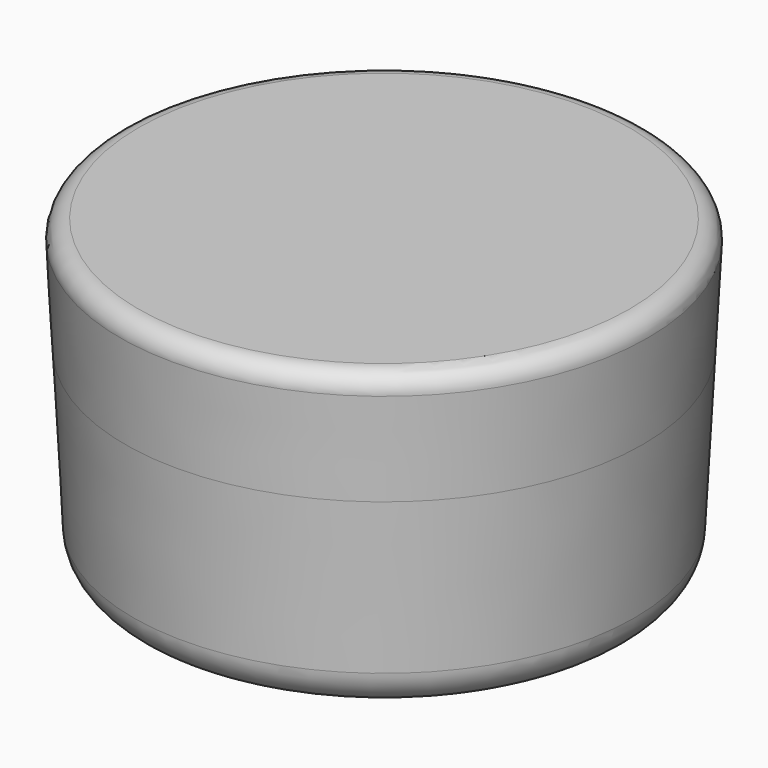
from build123d import *

# Parameters (mm, degrees)
F0_R     = 32.5
F1_DEPTH = 25
F1_TAPER = -3
F2_R     = 33.8101944821
F3_DEPTH = 15
F3_TAPER = -3
F4_R     = 2.4
F5_R     = 5


with BuildPart() as f1:
    # F0 (on Top) → F1 (new body)
    with BuildSketch(Plane.XY):
        Circle(F0_R)
    extrude(amount=F1_DEPTH, taper=F1_TAPER)

    # F5
    f5_edges = [f1.edges().sort_by_distance(p)[0] for p in [
        (-32.5, 0, 0),
    ]]
    fillet(f5_edges, radius=F5_R)


with BuildPart() as f3:
    # F2 (on face) → F3 (new body)
    with BuildSketch(Plane.XY.offset(25)):
        Circle(F2_R)
    extrude(amount=F3_DEPTH, taper=F3_TAPER)

    # F4
    f4_edges = [f3.edges().sort_by_distance(p)[0] for p in [
        (-34.596311, 0, 40),
    ]]
    fillet(f4_edges, radius=F4_R)


solid = Compound([f1.part, f3.part])
